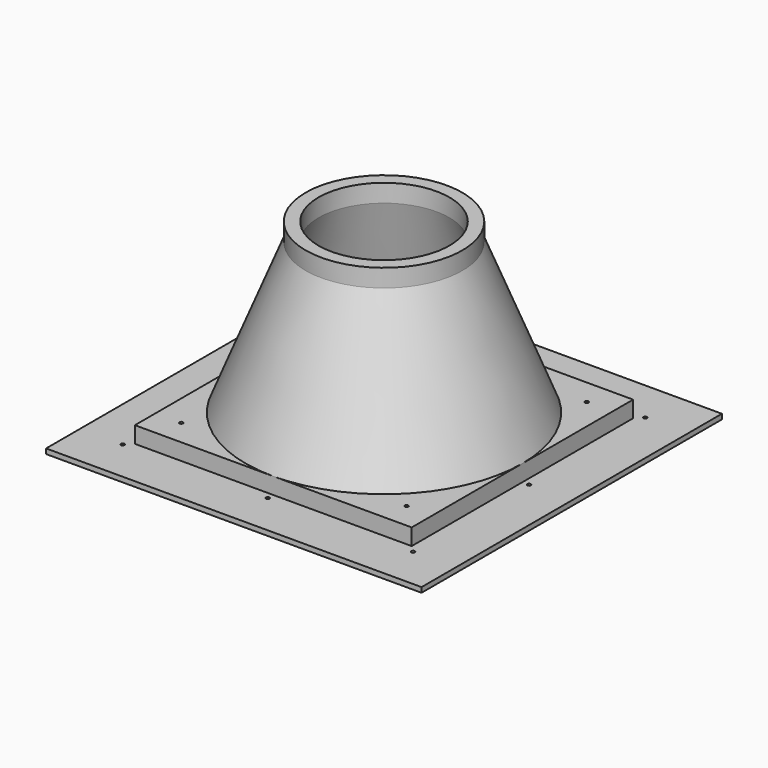
from build123d import *

# Parameters (mm, degrees)
F0_W      = 525
F0_H      = 525
F0_W_2    = 387
F0_H_2    = 387
F1_DEPTH  = 7
F2_DEPTH  = 30
F4_DEPTH  = 7
F7_DEPTH  = 25
F8_D      = 5
F9_D      = 5
F10_D     = 5
F11_D     = 5
F12_D     = 5
F13_R     = 2.5
F13_R_2   = 7.5
F14_DEPTH = 10


# Not quite as in the source:
# - a feature names something its author has since deleted; it is built from what else it names


with BuildPart() as f1:
    # F0 (on Top) → F1 (new body)
    with BuildSketch(Plane.XY):
        Rectangle(F0_W, F0_H)
        Rectangle(F0_W_2, F0_H_2, mode=Mode.SUBTRACT)
    extrude(amount=F1_DEPTH)

    # F0 (on Top) → F2 (join)
    with BuildSketch(Plane.XY):
        Rectangle(F0_W_2, F0_H_2)
        Polygon((-187.5, -6.596e-07), (-187.5, 187.5), (-6.149e-07, 187.5), (187.5, 187.5), (187.5, 0), (187.5, -187.5), (-6.893e-07, -187.5), (-187.5, -187.5), align=None, mode=Mode.SUBTRACT)
    extrude(amount=F2_DEPTH)

    # F3 (on face) → F4 (join)
    with BuildSketch(Plane.XY.offset(30)):
        with BuildLine():
            ThreePointArc((-187.5, 47.8121323515), (-136.8251621596, 136.8251621596), (-47.8121323515, 187.5))
            Line((-47.8121323515, 187.5), (-187.5, 187.5))
            Line((-187.5, 187.5), (-187.5, 47.8121323515))
        make_face()
        with BuildLine():
            ThreePointArc((-6.149e-07, 187.5), (132.5825212551, 132.5825216899), (187.5, 0))
            Line((187.5, 0), (187.5, 47.8121323515))
            ThreePointArc((187.5, 47.8121323515), (136.8251621596, 136.8251621596), (47.8121323515, 187.5))
            Line((47.8121323515, 187.5), (-6.149e-07, 187.5))
        make_face()
        with BuildLine():
            ThreePointArc((-187.5, -6.596e-07), (-132.5825219231, 132.5825210219), (-6.149e-07, 187.5))
            Line((-6.149e-07, 187.5), (-47.8121323515, 187.5))
            ThreePointArc((-47.8121323515, 187.5), (-136.8251621596, 136.8251621596), (-187.5, 47.8121323515))
            Line((-187.5, 47.8121323515), (-187.5, -6.596e-07))
        make_face()
        with BuildLine():
            Line((-47.8121323515, -187.5), (-6.893e-07, -187.5))
            ThreePointArc((-6.893e-07, -187.5), (-132.582521483, -132.582521462), (-187.5, -6.596e-07))
            Line((-187.5, -6.596e-07), (-187.5, -47.8121323515))
            ThreePointArc((-187.5, -47.8121323515), (-136.8251621596, -136.8251621596), (-47.8121323515, -187.5))
        make_face()
        with BuildLine():
            Line((187.5, -47.8121323515), (187.5, 0))
            ThreePointArc((187.5, 0), (132.5825212288, -132.5825217162), (-6.893e-07, -187.5))
            Line((-6.893e-07, -187.5), (47.8121323515, -187.5))
            ThreePointArc((47.8121323515, -187.5), (136.8251621596, -136.8251621596), (187.5, -47.8121323515))
        make_face()
        with BuildLine():
            ThreePointArc((47.8121323515, 187.5), (136.8251621596, 136.8251621596), (187.5, 47.8121323515))
            Line((187.5, 47.8121323515), (187.5, 187.5))
            Line((187.5, 187.5), (47.8121323515, 187.5))
        make_face()
        with BuildLine():
            Line((187.5, -187.5), (187.5, -47.8121323515))
            ThreePointArc((187.5, -47.8121323515), (136.8251621596, -136.8251621596), (47.8121323515, -187.5))
            Line((47.8121323515, -187.5), (187.5, -187.5))
        make_face()
        with BuildLine():
            Line((-187.5, -187.5), (-47.8121323515, -187.5))
            ThreePointArc((-47.8121323515, -187.5), (-136.8251621596, -136.8251621596), (-187.5, -47.8121323515))
            Line((-187.5, -47.8121323515), (-187.5, -187.5))
        make_face()
    extrude(amount=-F4_DEPTH)

    # F5 (on Front) → F6 (revolve)
    with BuildSketch(Plane.XZ):
        Polygon((-109.5, 240), (-193.5, 30), (-149.8333333333, 30), (-91.5, 240), align=None)
    revolve(axis=Axis((0, 0, 120), (0, 0, 1)))

    # F7 (add): a face of the model
    f7_faces = [f1.faces().sort_by_distance(p)[0] for p in [
        (94.5971277016, 0, 240),
    ]]
    extrude(f7_faces, amount=F7_DEPTH)

    # F8 (through all)
    with Locations(Plane(origin=(0, 0, 0), x_dir=(1, 0, 0), z_dir=(0, 0, -1))):
        with Locations((-157.5, -157.5)):
            Hole(F8_D / 2)

    # F9 (through all)
    with Locations(Plane(origin=(0, 0, 0), x_dir=(1, 0, 0), z_dir=(0, 0, -1))):
        with Locations((157.5, -157.5)):
            Hole(F9_D / 2)

    # F10 (through all)
    with Locations(Plane(origin=(0, 0, 0), x_dir=(1, 0, 0), z_dir=(0, 0, -1))):
        with Locations((-157.5, 157.5)):
            Hole(F10_D / 2)

    # F11 (through all)
    with Locations(Plane(origin=(0, 0, 0), x_dir=(1, 0, 0), z_dir=(0, 0, -1))):
        with Locations((157.5, 157.5)):
            Hole(F11_D / 2)

    # F12 (through all)
    with Locations(Plane(origin=(0, 0, 0), x_dir=(1, 0, 0), z_dir=(0, 0, -1))):
        with Locations((-203, -203), (0, -203), (203, -203), (203, 0), (203, 203), (0, 203), (-203, 203), (-203, 0)):
            Hole(F12_D / 2)

    # F13 (on face) → F14 (cut)
    with BuildSketch(Plane.XY.offset(30)):
        with Locations((157.5, -157.5)):
            Circle(F13_R)
        with Locations((-157.5, -157.5)):
            Circle(F13_R_2)
        with Locations((-157.5, 157.5)):
            Circle(F13_R_2)
        with Locations((157.5, 157.5)):
            Circle(F13_R_2)
    extrude(amount=F14_DEPTH, mode=Mode.SUBTRACT)


solid = f1.part
